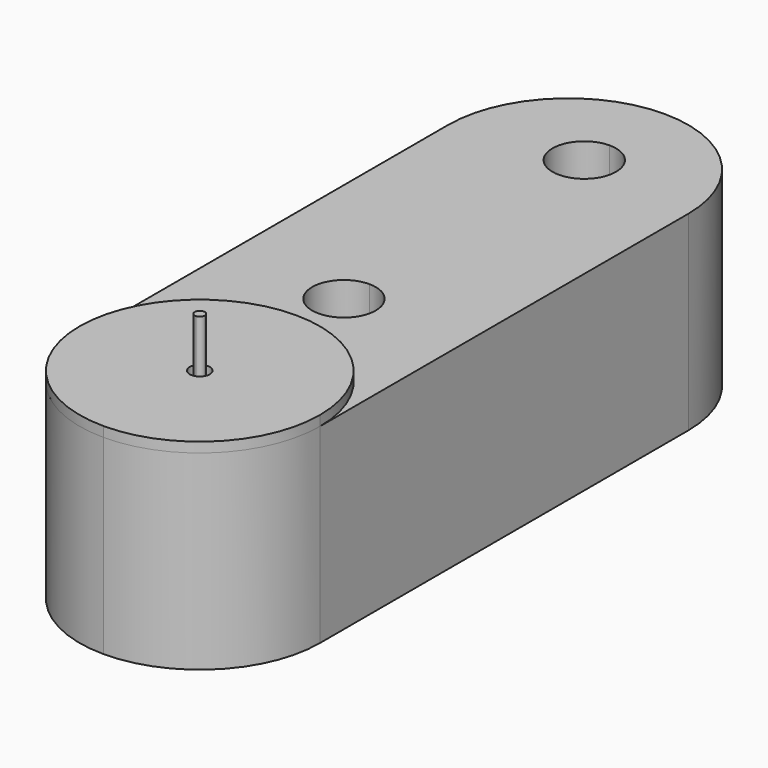
from build123d import *

# Parameters (mm, degrees)
F1_DEPTH      = 19.05
F2_R          = 1
F3_DEPTH      = 1
F5_DEPTH      = 6
F5_DEPTH_BACK = 25
F6_R          = 11.99999


# Not quite as in the source:
# - a fillet or chamfer is up to 0.001 mm smaller than in the source, because OpenCascade refuses the exact size


with BuildPart() as f1:
    # F0 (on Top) → F1 (new body)
    with BuildSketch(Plane.XY):
        with BuildLine():
            Line((12, -35), (12, 35))
            Line((12, 35), (0, 35))
            Line((0, 35), (0, 28.175))
            ThreePointArc((0, 28.175), (2.2450640303, 27.2450640303), (3.175, 25))
            ThreePointArc((3.175, 25), (2.2450640303, 22.7549359697), (0, 21.825))
            Line((0, 21.825), (0, -1.825))
            ThreePointArc((0, -1.825), (2.2450640303, -2.7549359697), (3.175, -5))
            ThreePointArc((3.175, -5), (2.2450640303, -7.2450640303), (0, -8.175))
            Line((0, -8.175), (0, -22.5))
            ThreePointArc((0, -22.5), (0.3535533906, -22.6464466094), (0.5, -23))
            ThreePointArc((0.5, -23), (0.3535533906, -23.3535533906), (0, -23.5))
            Line((0, -23.5), (0, -35))
            Line((0, -35), (12, -35))
        make_face()
        with BuildLine():
            Line((0, 28.175), (0, 35))
            Line((0, 35), (-12, 35))
            Line((-12, 35), (-12, -35))
            Line((-12, -35), (0, -35))
            Line((0, -35), (0, -23.5))
            ThreePointArc((0, -23.5), (-0.5, -23), (0, -22.5))
            Line((0, -22.5), (0, -8.175))
            ThreePointArc((0, -8.175), (-3.175, -5), (0, -1.825))
            Line((0, -1.825), (0, 21.825))
            ThreePointArc((0, 21.825), (-3.175, 25), (0, 28.175))
        make_face()
    extrude(amount=F1_DEPTH)

    # F6 (radius 12 in the source; OpenCascade refuses exactly that, so slightly less here)
    f6_edges = [f1.edges().sort_by_distance(p)[0] for p in [
        (-12, 35, 9.525),
        (12, 35, 9.525),
        (12, -35, 9.525),
        (-12, -35, 9.525),
    ]]
    fillet(f6_edges, radius=F6_R)


with BuildPart() as f3:
    # F2 (on face) → F3 (new body)
    with BuildSketch(Plane.XY.offset(19.05)):
        with BuildLine():
            ThreePointArc((0, -35), (8.4852813742, -31.4852813742), (12, -23))
            ThreePointArc((12, -23), (-5.29e-08, -11), (-12, -23.0000001058))
            ThreePointArc((-12, -23.0000001058), (-8.4852813368, -31.4852814116), (0, -35))
        make_face()
        with Locations((0, -23)):
            Circle(F2_R, mode=Mode.SUBTRACT)
    extrude(amount=F3_DEPTH)


with BuildPart() as f5:
    # F4 (on face) → F5 (new body, two sides)
    with BuildSketch(Plane.XY.offset(19.05)) as f5_sk:
        with BuildLine():
            ThreePointArc((0, -23.5), (0.3535533906, -23.3535533906), (0.5, -23))
            ThreePointArc((0.5, -23), (-0.3535533906, -22.6464466094), (0, -23.5))
        make_face()
    extrude(amount=F5_DEPTH)
    extrude(f5_sk.sketch, amount=-F5_DEPTH_BACK)


solid = Compound([f1.part, f3.part, f5.part])
